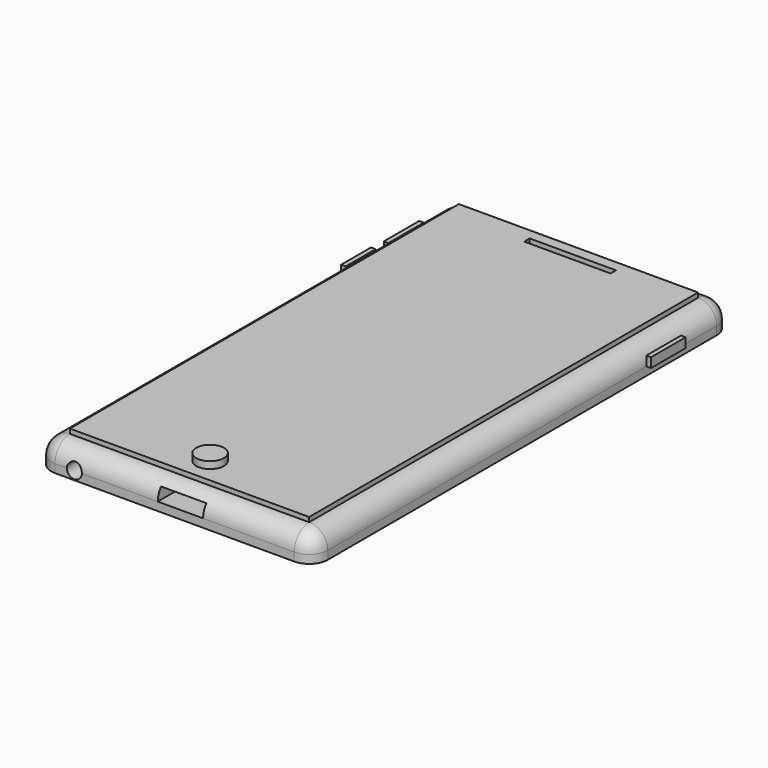
from build123d import *

# Parameters (mm, degrees)
F0_W      = 75.4051078111
F0_H      = 142.7516564727
F1_DEPTH  = 7.366
F2_F1_R   = 5.08
F2_F2_R   = 5.08
F2_F3_R   = 5.08
F2_F4_R   = 5.08
F3_W      = 12.3756472021
F3_H      = 3.1823093913
F4_DEPTH  = 6.35
F5_R      = 2.046755254
F6_DEPTH  = 6.35
F7_W      = 65.2451078111
F7_H      = 132.5916564727
F8_DEPTH  = 1.27
F9_W      = 11.800032109
F9_H      = 2.6066980235
F10_DEPTH = 1.27
F11_R     = 3.7854916829
F12_DEPTH = 1.905
F13_W     = 23.5232524574
F13_H     = 1.857098192
F14_DEPTH = 6.35
F15_W     = 12.0711438358
F15_H     = 2.5115047491
F16_DEPTH = 1.27
F17_W     = 10.2140437812
F17_H     = 2.8210214249
F18_DEPTH = 1.27
F20_DEPTH = 1.27


with BuildPart() as f1:
    # F0 (on Top) → F1 (new body)
    with BuildSketch(Plane.XY):
        with Locations((-26.1903246865, -3.4536682069)):
            Rectangle(F0_W, F0_H)
    extrude(amount=F1_DEPTH)

    # F2: fillet of radius 5.08 on 8 edges, made by hand

    # F2_f1
    f2_f1_edges = [f1.edges().sort_by_distance(p)[0] for p in [
        (11.5122292191, 67.9221600294, 3.683),
    ]]
    fillet(f2_f1_edges, radius=F2_F1_R)

    # F2_f2
    f2_f2_edges = [f1.edges().sort_by_distance(p)[0] for p in [
        (-63.892878592, 67.9221600294, 3.683),
    ]]
    fillet(f2_f2_edges, radius=F2_F2_R)

    # F2_f3
    f2_f3_edges = [f1.edges().sort_by_distance(p)[0] for p in [
        (-26.1903246865, 67.9221600294, 7.366),
    ]]
    fillet(f2_f3_edges, radius=F2_F3_R)

    # F2_f4
    f2_f4_edges = [f1.edges().sort_by_distance(p)[0] for p in [
        (-63.892878592, -74.8294964433, 1.143),
    ]]
    fillet(f2_f4_edges, radius=F2_F4_R)

    # F3 (on face) → F4 (cut)
    with BuildSketch(Plane.XZ.offset(74.8294964433)):
        with Locations((-24.6073929593, 3.8771546956)):
            Rectangle(F3_W, F3_H)
    extrude(amount=-F4_DEPTH, mode=Mode.SUBTRACT)

    # F5 (on face) → F6 (cut)
    with BuildSketch(Plane.XZ.offset(74.8294964433)):
        with Locations((-53.5318702459, 2.286)):
            Circle(F5_R)
    extrude(amount=-F6_DEPTH, mode=Mode.SUBTRACT)


with BuildPart() as f8:
    # F7 (on face) → F8 (new body)
    with BuildSketch(Plane.XY.offset(7.366)):
        with Locations((-26.1903246865, -3.4536682069)):
            Rectangle(F7_W, F7_H)
    extrude(amount=F8_DEPTH)

    # F13 (on face) → F14 (cut)
    with BuildSketch(Plane.XY.offset(8.636)):
        with Locations((-25.3803487867, 58.9628834277)):
            Rectangle(F13_W, F13_H)
    extrude(amount=-F14_DEPTH, mode=Mode.SUBTRACT)


with BuildPart() as f10:
    # F9 (on face) → F10 (new body)
    with BuildSketch(Plane.YZ.offset(11.5122292191)):
        with Locations((44.7537954897, 3.5893490117)):
            Rectangle(F9_W, F9_H)
    extrude(amount=F10_DEPTH)


with BuildPart() as f12:
    # F11 (on face) → F12 (new body)
    with BuildSketch(Plane.XY.offset(8.636)):
        with Locations((-26.1903246865, -62.7416521311)):
            Circle(F11_R)
    extrude(amount=F12_DEPTH)


with BuildPart() as f16:
    # F15 (on face) → F16 (new body)
    with BuildSketch(Plane(origin=(-63.892878592, 0, 0), x_dir=(0, -1, 0), z_dir=(-1, 0, 0))):
        with Locations((-51.2249711901, 3.5417523746)):
            Rectangle(F15_W, F15_H)
    extrude(amount=F16_DEPTH)


with BuildPart() as f18:
    # F17 (on face) → F18 (new body)
    with BuildSketch(Plane(origin=(-63.892878592, 0, 0), x_dir=(0, -1, 0), z_dir=(-1, 0, 0))):
        with Locations((-35.7491495088, 3.6965107125)):
            Rectangle(F17_W, F17_H)
    extrude(amount=F18_DEPTH)


with BuildPart() as f20:
    # F19 (on face) → F20 (new body)
    with BuildSketch(Plane(origin=(0, 0, 0), x_dir=(1, 0, 0), z_dir=(0, 0, -1))):
        with BuildLine():
            add(Edge.make_bspline(
                [(-26.9279293716, -37.296731025), (-26.1590478095, -37.8796180067), (-27.2405076799, -41.610190349), (-33.6150642057, -44.8689171286), (-32.8227501646, -38.2996334195), (-27.8316461583, -36.6116258331), (-26.9279293716, -37.296731025)],
                knots=[0, 0, 0, 0, 0.2291805231, 0.4943005153, 0.7306291422, 1, 1, 1, 1], degree=3))
        make_face()
    extrude(amount=F20_DEPTH)


with BuildPart() as f20b:
    # F19 (on face) → F20, piece 2 (new body)
    with BuildSketch(Plane(origin=(0, 0, 0), x_dir=(1, 0, 0), z_dir=(0, 0, -1))):
        with BuildLine():
            add(Edge.make_bspline(
                [(-18.5709875077, -34.8206013441), (-16.9933307569, -34.4069620178), (-14.1792039609, -33.0899210778), (-13.7777924329, -27.883110785), (-14.272988719, -21.6169154673), (-16.351813669, -16.762216435), (-21.0363385209, -9.9297464764), (-26.8947206756, -14.9211673759), (-32.2389811264, -11.130286541), (-36.3725185757, -14.0623640639), (-39.5224923345, -18.8545713408), (-37.2114139136, -21.0298104682), (-34.5153706863, -27.1103805858), (-36.2968935413, -29.969179565), (-39.0716980584, -31.7151857926), (-37.5791604466, -35.9829722305), (-31.7963960221, -34.5523022934), (-29.4355823464, -34.9774247098), (-26.8124785552, -32.318446701), (-23.9298221224, -35.599274808), (-20.3161966458, -35.2781705408), (-18.5709875077, -34.8206013441)],
                knots=[0, 0, 0, 0, 0.0520581477, 0.10668462, 0.1693019503, 0.2291883895, 0.2935167278, 0.3538845551, 0.4122524688, 0.4659202448, 0.522004706, 0.5637754073, 0.6266239453, 0.6704560449, 0.7128646393, 0.7566967388, 0.814283655, 0.8539413629, 0.8957120516, 0.9424131041, 1, 1, 1, 1], degree=3))
        make_face()
    extrude(amount=F20_DEPTH)


solid = Compound([f1.part, f8.part, f10.part, f12.part, f16.part, f18.part, f20.part, f20b.part])
